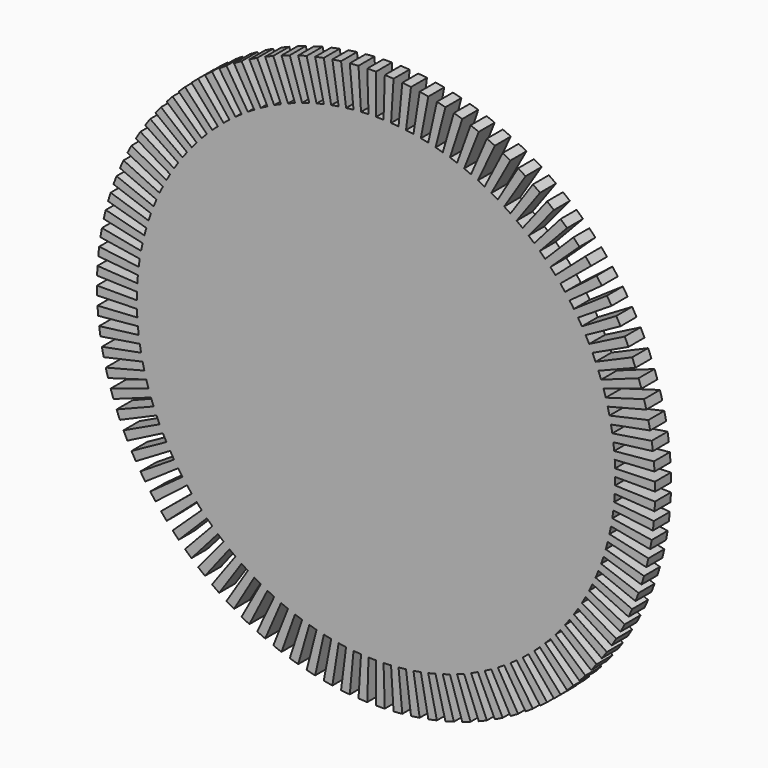
from build123d import *

# Parameters (mm, degrees)
F1_DEPTH        = 1.5875
F2_DEPTH        = 25.4
F2_COPIES_COUNT = 100


# Not quite as in the source:
# - a pattern or mirror of a feature is missing from the dataset's text; its kind, count and spacing are read off the source's solid


with BuildPart() as f1:
    # F0 (on Front) → F1 (new body)
    with BuildSketch(Plane.XZ):
        with BuildLine():
            ThreePointArc((0, 22.225), (-15.7154482119, -15.7154482119), (22.225, 0))
            ThreePointArc((22.225, 0), (15.9603569678, 15.4666619043), (0.6981041205, 22.2140333041))
            Line((0.6981041205, 22.2140333041), (0.5983749604, 19.040599975))
            ThreePointArc((0.5983749604, 19.040599975), (13.6803059724, 13.2571387751), (19.05, 0))
            ThreePointArc((19.05, 0), (-13.4703841816, -13.4703841816), (0, 19.05))
            Line((0, 19.05), (0, 22.225))
        make_face()
        with BuildLine():
            ThreePointArc((19.05, 0), (13.6803059724, 13.2571387751), (0.5983749604, 19.040599975))
            ThreePointArc((0.5983749604, 19.040599975), (0.2992243948, 19.0476498488), (0, 19.05))
            ThreePointArc((0, 19.05), (-13.4703841816, -13.4703841816), (19.05, 0))
        make_face()
        with BuildLine():
            Line((0.5983749604, 19.040599975), (0.6981041205, 22.2140333041))
            ThreePointArc((0.6981041205, 22.2140333041), (0.3490951273, 22.2222581569), (0, 22.225))
            Line((0, 22.225), (0, 19.05))
            ThreePointArc((0, 19.05), (0.2992243948, 19.0476498488), (0.5983749604, 19.040599975))
        make_face()
    extrude(amount=-F1_DEPTH)

    # F0 (on Front) → F2 (cut)
    with BuildSketch(Plane.XZ):
        with BuildLine():
            Line((0.5983749604, 19.040599975), (0.6981041205, 22.2140333041))
            ThreePointArc((0.6981041205, 22.2140333041), (0.3490951273, 22.2222581569), (0, 22.225))
            Line((0, 22.225), (0, 19.05))
            ThreePointArc((0, 19.05), (0.2992243948, 19.0476498488), (0.5983749604, 19.040599975))
        make_face()
    f2 = extrude(amount=-F2_DEPTH, mode=Mode.SUBTRACT)

    # F2_copies: F2 ×100 about axis
    f2_copies_axis = Axis((0, 0, 0), (0, 1, 0))
    for i in range(1, F2_COPIES_COUNT):
        add(f2.rotate(f2_copies_axis, i * 360 / F2_COPIES_COUNT), mode=Mode.SUBTRACT)


solid = f1.part
